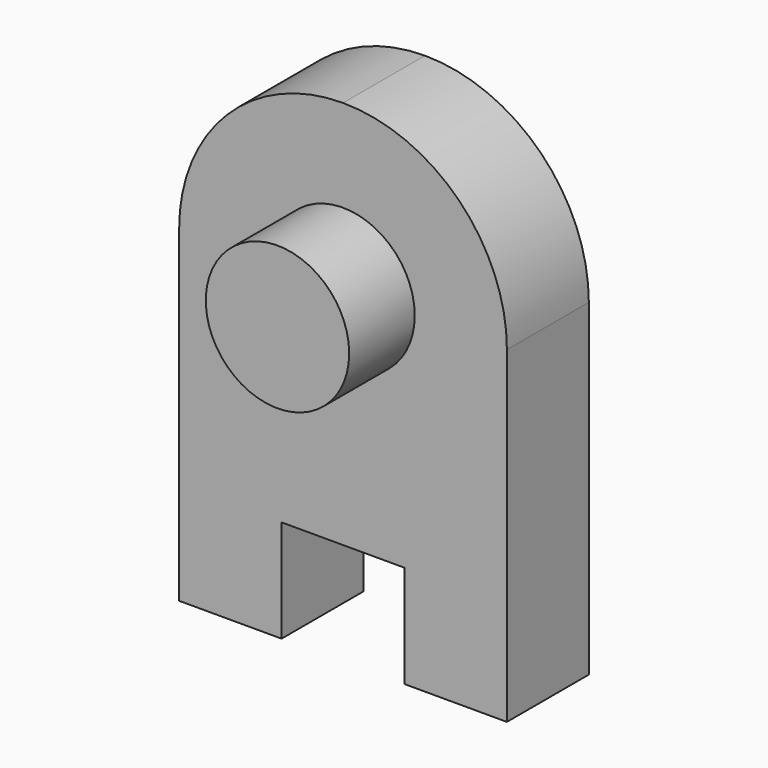
from build123d import *

# Parameters (mm, degrees)
F0_W     = 80
F0_H     = 120
F1_DEPTH = 25
F2_R     = 39.99999
F3_W     = 30
F3_H     = 50
F4_DEPTH = 25.001
F5_R     = 17.5
F6_DEPTH = 20


# Not quite as in the source:
# - a fillet or chamfer is up to 0.001 mm smaller than in the source, because OpenCascade refuses the exact size


with BuildPart() as f1:
    # F0 (on Front) → F1 (new body)
    with BuildSketch(Plane.XZ):
        Rectangle(F0_W, F0_H)
    extrude(amount=F1_DEPTH)

    # F2 (radius 40 in the source; OpenCascade refuses exactly that, so slightly less here)
    f2_edges = [f1.edges().sort_by_distance(p)[0] for p in [
        (40, -12.5, 60),
        (-40, -12.5, 60),
    ]]
    fillet(f2_edges, radius=F2_R)

    # F3 (on face) → F4 (cut, through all)
    with BuildSketch(Plane.XZ.offset(25)):
        with Locations((0, -60)):
            Rectangle(F3_W, F3_H)
    extrude(amount=-F4_DEPTH, mode=Mode.SUBTRACT)

    # F5 (on face) → F6 (join)
    with BuildSketch(Plane.XZ.offset(25)):
        with Locations((0, 20)):
            Circle(F5_R)
    extrude(amount=F6_DEPTH)


solid = f1.part
